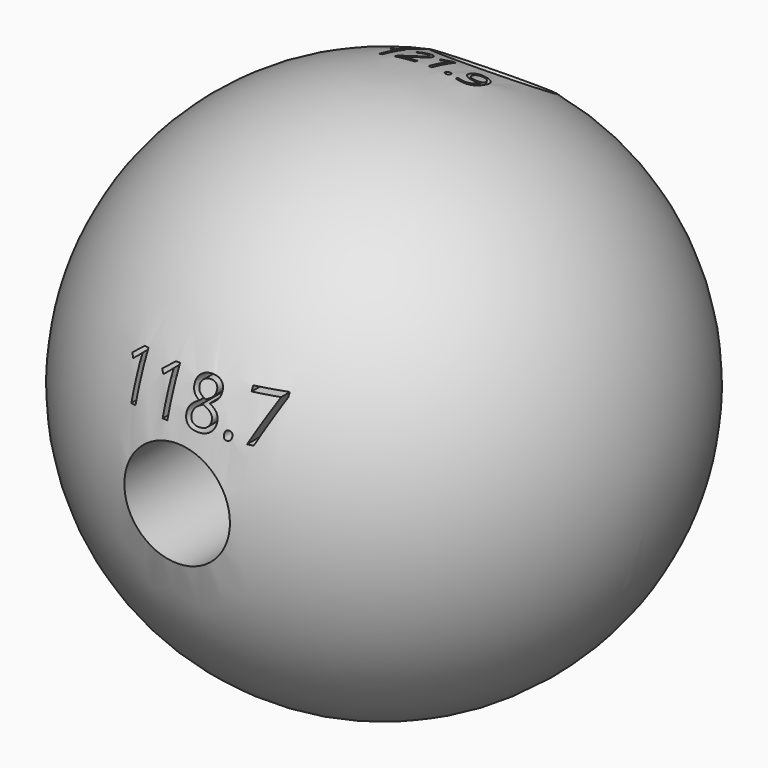
from build123d import *

# Parameters (mm, degrees)
F4_R          = 3.175
F5_DEPTH      = 25.4
F7_ANGLE      = 119.3
F9_ANGLE      = -121.9
F11_TEXT_SIZE = 3.7115979164
F12_DEPTH     = 10.16
F14_TEXT_SIZE = 2.4966775931
F15_DEPTH     = 10.16
F17_TEXT_SIZE = 4.8943083837
F18_DEPTH     = 10.16


# Not quite as in the source:
# - Text() gives the source's letters only with a copy of the font that has no kerning and outlines rounded to 1/6400 em; it was checked with that copy


with BuildPart() as f2:
    # F0 (on Front) → F2 (revolve)
    with BuildSketch(Plane.XZ):
        with BuildLine():
            Line((1.6591942403, 0), (-15.875, 0))
            ThreePointArc((-15.875, 0), (0, -15.875), (15.875, 0))
            Line((15.875, 0), (1.6591942403, 0))
        make_face()
    revolve(axis=Axis((0, 0, 0), (1, 0, 0)))

    # F11 (on offset) → F12 (cut)
    with BuildSketch(Plane.XZ.offset(17.78)):
        with Locations((-4.1894102469, 4.0581328794)):
            Text('118.7', F11_TEXT_SIZE, font='Open Sans', text_align=(TextAlign.LEFT, TextAlign.BOTTOM))
    extrude(amount=-F12_DEPTH, mode=Mode.SUBTRACT)

    # F14 (on offset) → F15 (cut)
    with BuildSketch(Plane(origin=(0, 9.2614102543, 14.8790777974), x_dir=(1, 0, 0), z_dir=(0, 0.5284383347, 0.8489716876))):
        with Locations((-3.4555724123, -5.4499777034)):
            Text('121.9', F14_TEXT_SIZE, font='Open Sans', text_align=(TextAlign.LEFT, TextAlign.BOTTOM))
    extrude(amount=-F15_DEPTH, mode=Mode.SUBTRACT)

    # F17 (on offset) → F18 (cut)
    with BuildSketch(Plane(origin=(0, 8.5769168494, -15.2838860686), x_dir=(1, 0, 0), z_dir=(0, 0.4893824517, -0.8720692724))):
        with Locations((-5.8323929552, -8.3835176192)):
            Text('119.3', F17_TEXT_SIZE, font='Open Sans', text_align=(TextAlign.LEFT, TextAlign.BOTTOM))
    extrude(amount=-F18_DEPTH, mode=Mode.SUBTRACT)


with BuildPart() as f5:
    # F4 (on offset) → F5 (new body)
    with BuildSketch(Plane.XZ.offset(6.35)):
        Circle(F4_R)
    extrude(amount=F5_DEPTH)


with BuildPart() as f7_1:
    # F7: copy of F5
    add(f5.part.rotate(Axis((5.4384693503, 0, 0), (1, 0, 0)), F7_ANGLE))


with BuildPart() as f9_1:
    # F9: copy of F5
    add(f5.part.rotate(Axis((-2.7653239667, 0, 0), (1, 0, 0)), F9_ANGLE))


with BuildPart() as f2_1:
    add(f2.part)

    # F19: cut F5, F9_1, F7_1
    add(f5.part, mode=Mode.SUBTRACT)
    add(f9_1.part, mode=Mode.SUBTRACT)
    add(f7_1.part, mode=Mode.SUBTRACT)


solid = f2_1.part
